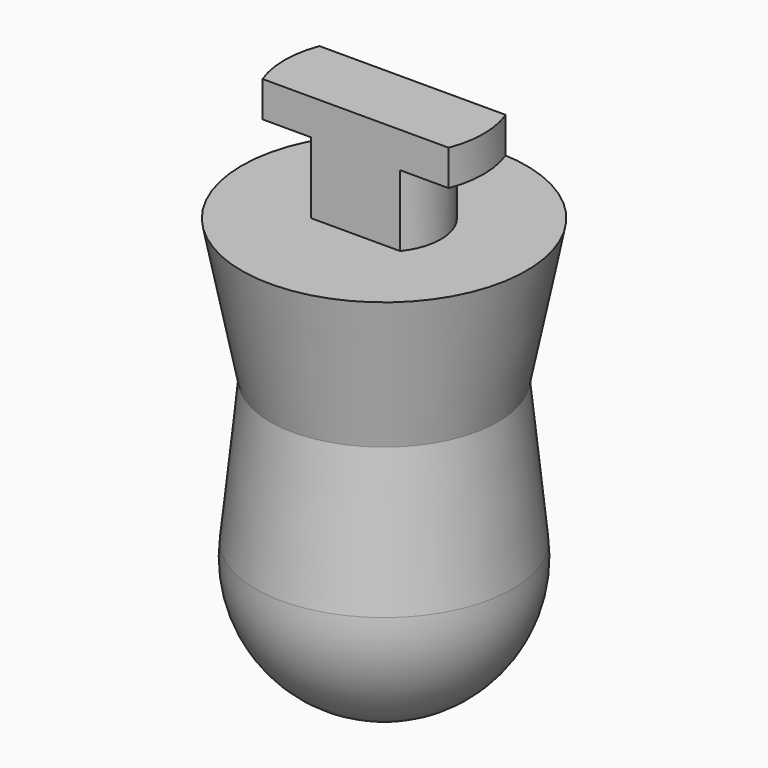
from build123d import *

# Parameters (mm, degrees)
F3_DEPTH = 9.525


with BuildPart() as f1:
    # F0 (on Front) → F1 (revolve)
    with BuildSketch(Plane.XZ):
        Polygon((0, -12.7), (0, 0), (-5.08, 0), (-12.7, 0), (-10.16, -12.7), align=None)
        Polygon((-5.08, 0), (0, 0), (0, 9.525), (-8.89, 9.525), (-8.89, 6.35), (-5.08, 6.35), align=None)
        Polygon((0, -25.4), (0, -12.7), (-10.16, -12.7), (-11.4633519053, -25.4), align=None)
        with BuildLine():
            Line((0, -38.1), (0, -25.4))
            Line((0, -25.4), (-11.4633519053, -25.4))
            ThreePointArc((-11.4633519053, -25.4), (-8.5542158744, -34.2976982984), (0, -38.1))
        make_face()
    revolve(axis=Axis((0, 0, -19.05), (0, 0, -1)))

    # F2 (on face) → F3 (cut, through all)
    with BuildSketch(Plane.XY.offset(9.525)):
        with BuildLine():
            ThreePointArc((8.3037024874, 3.175), (0, 8.89), (-8.3037024874, 3.175))
            Line((-8.3037024874, 3.175), (8.3037024874, 3.175))
        make_face()
        with BuildLine():
            Line((8.3037024874, -3.175), (-8.3037024874, -3.175))
            ThreePointArc((-8.3037024874, -3.175), (0, -8.89), (8.3037024874, -3.175))
        make_face()
        with BuildLine():
            ThreePointArc((10.9695693512, 3.175), (0, 11.4198107144), (-10.9695693512, 3.175))
            Line((-10.9695693512, 3.175), (-8.3037024874, 3.175))
            ThreePointArc((-8.3037024874, 3.175), (0, 8.89), (8.3037024874, 3.175))
            Line((8.3037024874, 3.175), (10.9695693512, 3.175))
        make_face()
        with BuildLine():
            Line((-8.3037024874, -3.175), (-10.9695693512, -3.175))
            ThreePointArc((-10.9695693512, -3.175), (0, -11.4198107144), (10.9695693512, -3.175))
            Line((10.9695693512, -3.175), (8.3037024874, -3.175))
            ThreePointArc((8.3037024874, -3.175), (0, -8.89), (-8.3037024874, -3.175))
        make_face()
        with BuildLine():
            Line((-8.3037024874, 3.175), (-10.9695693512, 3.175))
            ThreePointArc((-10.9695693512, 3.175), (-11.4198107144, 0), (-10.9695693512, -3.175))
            Line((-10.9695693512, -3.175), (-8.3037024874, -3.175))
            ThreePointArc((-8.3037024874, -3.175), (-8.89, 0), (-8.3037024874, 3.175))
        make_face()
        with BuildLine():
            ThreePointArc((11.4198107144, 0), (11.3066901072, 1.6033825405), (10.9695693512, 3.175))
            Line((10.9695693512, 3.175), (8.3037024874, 3.175))
            ThreePointArc((8.3037024874, 3.175), (8.7421969525, 1.6143396307), (8.89, 0))
            ThreePointArc((8.89, 0), (8.7421969525, -1.6143396307), (8.3037024874, -3.175))
            Line((8.3037024874, -3.175), (10.9695693512, -3.175))
            ThreePointArc((10.9695693512, -3.175), (11.3066901072, -1.6033825405), (11.4198107144, 0))
        make_face()
    extrude(amount=-F3_DEPTH, mode=Mode.SUBTRACT)


solid = f1.part
